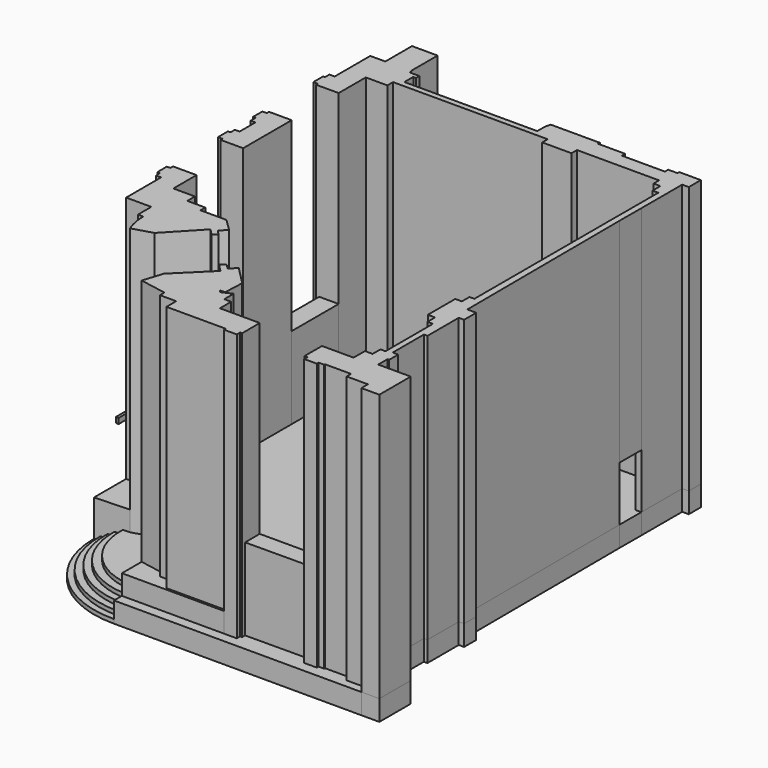
from build123d import *

# Parameters (mm, degrees)
F1_DEPTH      = 9800
F0_W          = 4864.5615577698
F0_H          = 206.8319521715
F2_START      = 2000
F2_DEPTH      = 7800
F3_DEPTH      = 730
F3_DEPTH_BACK = 750
F4_DEPTH      = 2800
F0_W_2        = 366.9002056122
F0_H_2        = 2132.168845481
F0_W_3        = 154.331445694
F0_W_4        = 212.5687599182
F0_W_5        = 342.2532081604
F0_H_3        = 2150.8503360921
F0_W_6        = 172.8549003601
F0_W_7        = 200.4117965698
F5_DEPTH      = 750
F6_START      = -150
F6_DEPTH      = 600
F7_START      = -300
F7_DEPTH      = 450
F8_START      = -450
F8_DEPTH      = 300
F9_START      = -600
F9_DEPTH      = 150
F10_DEPTH     = 3000
F12_W         = 7000
F12_H         = 200
F13_DEPTH     = 100
F14_R         = 253.1505474525
F15_DEPTH     = 1800


with BuildPart() as f1:
    # F0 (on Top) → F1 (new body)
    with BuildSketch(Plane.XY):
        with BuildLine():
            Line((8390.4028525727, 2896.5206632115), (7940.039693393, 3339.2489442326))
            Line((7940.039693393, 3339.2489442326), (6987.7205481903, 3339.2489442326))
            Line((6987.7205481903, 3339.2489442326), (6987.7205481903, 3558.5393704603))
            Line((6987.7205481903, 3558.5393704603), (6329.7600746155, 3558.5393704603))
            Line((6329.7600746155, 3558.5393704603), (6329.7600746155, 3909.2600144575))
            Line((6329.7600746155, 3909.2600144575), (5538.1336212158, 3909.2600144575))
            Line((5538.1336212158, 3909.2600144575), (5538.1336212158, 4971.1712833412))
            Line((5538.1336212158, 4971.1712833412), (5171.2334156036, 4971.1712833412))
            Line((5171.2334156036, 4971.1712833412), (5016.9019699097, 4971.1712833412))
            Line((5016.9019699097, 4971.1712833412), (4804.3332099915, 4971.1712833412))
            Line((4804.3332099915, 4971.1712833412), (4676.3634681702, 4971.1712833412))
            Line((4676.3634681702, 4971.1712833412), (4676.3634681702, 4850.8997164537))
            Line((4676.3634681702, 4850.8997164537), (4546.0958480835, 4850.8997164537))
            Line((4546.0958480835, 4850.8997164537), (4546.0958480835, 4420.0390811927))
            Line((4546.0958480835, 4420.0390811927), (4644.8583602905, 4420.0390811927))
            Line((4644.8583602905, 4420.0390811927), (4644.8583602905, 4229.7711372375))
            Line((4644.8583602905, 4229.7711372375), (4835.2494239807, 4229.7711372375))
            Line((4835.2494239807, 4229.7711372375), (4835.2494239807, 2626.4770030975))
            Line((4835.2494239807, 2626.4770030975), (5757.143497467, 2626.4770030975))
            Line((5757.143497467, 2626.4770030975), (5757.143497467, 2012.3040676117))
            Line((5757.143497467, 2012.3040676117), (5947.5092887878, 2012.3040676117))
            ThreePointArc((5947.5092887878, 2012.3040676117), (5992.5931204612, 1601.8080349278), (6110.9477729288, 1206.1671359211))
            Line((6110.9477729288, 1206.1671359211), (6839.3669128418, 1424.0067005157))
            Line((6839.3669128418, 1424.0067005157), (7948.8120079041, 2597.5522994995))
            Line((7948.8120079041, 2597.5522994995), (8010.4625259152, 2533.099484609))
            Line((8010.4625259152, 2533.099484609), (8155.1715442271, 2671.5168051709))
            Line((8155.1715442271, 2671.5168051709), (8390.4028525727, 2896.5206632115))
        make_face()
        Polygon((8318.0811700354, 2501.2021947697), (8155.1715442271, 2671.5168051709), (8010.4625259152, 2533.099484609), (8175.5933624414, 2360.4626993445), align=None)
    extrude(amount=F1_DEPTH)


with BuildPart() as f1b:
    # F0 (on Top) → F1, piece 2 (new body)
    with BuildSketch(Plane.XY):
        Polygon((5171.2334156036, 7103.3401288221), (5538.1336212158, 7103.3401288221), (5538.1336212158, 9326.2376584242), (5195.8804130554, 9326.2376584242), (5023.0255126953, 9326.2376584242), (4822.6137161255, 9326.2376584242), (4706.4251899719, 9326.2376584242), (4706.4251899719, 9225.9361946481), (4546.0958480835, 9225.9361946481), (4546.0958480835, 8795.1182157243), (4640.9873962402, 8795.1182157243), (4640.9873962402, 8570.7567960466), (4814.5852088928, 8570.7567960466), (4814.5852088928, 7846.2518483842), (4639.1639709473, 7846.2518483842), (4639.1639709473, 7645.8400518144), (4546.0958480835, 7645.8400518144), (4546.0958480835, 7191.3041867445), (4706.4251899719, 7191.3041867445), (4706.4251899719, 7103.3401288221), (4804.3332099915, 7103.3401288221), (5016.9019699097, 7103.3401288221), align=None)
    extrude(amount=F1_DEPTH)


with BuildPart() as f1c:
    # F0 (on Top) → F1, piece 3 (new body)
    with BuildSketch(Plane.XY):
        Polygon((5195.8804130554, 11477.0879945163), (5538.1336212158, 11477.0879945163), (5538.1336212158, 12718.5888089369), (6328.5875320435, 12718.5888089369), (6328.5875320435, 12979.1240491102), (6579.1020393372, 12979.1240491102), (6579.1020393372, 13185.9560012817), (6579.1020393372, 13590.3796948622), (6679.3084144592, 13590.3796948622), (6679.3084144592, 13743.2192050389), (6323.81772995, 13743.2192050389), (6323.81772995, 13838.4149753025), (6296.2608337402, 13838.4149753025), (6296.2608337402, 15059.0704165867), (5357.4075698853, 15059.0704165867), (5357.4075698853, 13838.4149753025), (4806.2753677368, 13838.4149753025), (4806.2753677368, 12207.3677264622), (4616.2400245667, 12207.3677264622), (4616.2400245667, 12006.9559298924), (4546.0958480835, 12006.9559298924), (4546.0958480835, 11556.0431338342), (4706.4251899719, 11556.0431338342), (4706.4251899719, 11477.0879945163), (4822.6137161255, 11477.0879945163), (5023.0255126953, 11477.0879945163), align=None)
        with Locations((9011.382818222, 13082.540025196)):
            Rectangle(F0_W, F0_H)
        Polygon((11443.6635971069, 13185.9560012817), (11443.6635971069, 12979.1240491102), (11992.54322052, 12979.1240491102), (11992.54322052, 12727.0231246948), (13064.7459030151, 12727.0231246948), (13064.7459030151, 12979.1240491102), (16070.9228515625, 12979.1240491102), (16070.9228515625, 12727.0231246948), (16321.4359283447, 12727.0231246948), (16321.4359283447, 12366.2815093994), (16531.867980957, 12366.2815093994), (16531.867980957, 11314.1202926636), (16752.3212432861, 11314.1202926636), (16752.3212432861, 13185.9560012817), (16992.8150177002, 13185.9560012817), (16992.8150177002, 13739.1023635864), (16201.1890411377, 13739.1023635864), (16201.1890411377, 13658.9374542236), (15860.4898452759, 13658.9374542236), (15860.4898452759, 13508.6288452148), (14287.257194519, 13508.6288452148), (14287.257194519, 13658.9374542236), (13295.2194213867, 13658.9374542236), (13295.2194213867, 13739.1023635864), (11495.4862594604, 13739.1023635864), (11443.6635971069, 13556.6558837891), align=None)
    extrude(amount=F1_DEPTH)



with BuildPart() as f1d:
    # F0 (on Top) → F1, piece 4 (new body)
    with BuildSketch(Plane.XY):
        Polygon((17458.3015441895, -2084.8836898804), (17458.3015441895, -2384.4513893127), (18116.828918457, -2384.4513893127), (18116.828918457, -946.4971423149), (16924.3793487549, -946.4971423149), (16924.3793487549, -515.6118869781), (16984.5027923584, -515.6118869781), (16984.5027923584, -104.7678515315), (16784.0919494629, -104.7678515315), (16784.0919494629, 1320.7347393036), (16914.1807556152, 1320.7347393036), (16914.1807556152, 2753.9772987366), (17110.4774475098, 2753.9772987366), (17110.4774475098, 3310.1196289062), (16784.0919494629, 3310.1196289062), (16749.4583129883, 10318.6321258545), (16529.0050506592, 10318.6321258545), (16529.0050506592, 3949.7368335724), (16348.3219146729, 3949.7368335724), (16348.3219146729, 3602.5412082672), (16107.4104309082, 3602.5412082672), (16107.4104309082, 2348.3486175537), (16371.5972900391, 2348.3486175537), (16371.5972900391, 2000.5106925964), (16571.7658996582, 2000.5106925964), (16571.7658996582, -172.0592528582), (16387.3424530029, -172.0592528582), (16387.3424530029, -531.3978791237), (16107.4104309082, -531.3978791237), (16107.4104309082, -1052.1912574768), (14950.7637023926, -1052.1912574768), (14950.7637023926, -1344.4619244273), (14950.7637023926, -1511.5863084793), (14950.7637023926, -1712.9493697641), (14950.7637023926, -1860.01932621), (15058.1789016724, -1860.01932621), (15058.1789016724, -1999.9604225159), (15524.05834198, -1999.9604225159), (15524.05834198, -1918.4757471085), (15724.2269515991, -1918.4757471085), (15724.2269515991, -1883.047580719), (16678.1482696533, -1883.047580719), (16678.1482696533, -2084.8836898804), align=None)
    extrude(amount=F1_DEPTH)


with BuildPart() as f1e:
    # F0 (on Top) → F1, piece 5 (new body)
    with BuildSketch(Plane.XY):
        Polygon((9779.6468734741, 762.6244425774), (8624.6900558472, -378.161162138), (8390.8643722534, -1107.9804897308), (9367.6653263956, -1285.0561902172), (9368.6809539795, -1490.580049064), (9961.6676352145, -1490.580049064), (9963.8738632202, -1937.0355219255), (12124.6039412744, -1937.0355219255), (12124.9885559082, -2014.866692479), (12600.4909252113, -2014.866692479), (12599.7257232666, -1860.01932621), (12674.5738235881, -1860.01932621), (12673.9026556998, -1724.2008268784), (12672.8519885372, -1511.5863084793), (12672.0817630936, -1355.7223797609), (12670.581817627, -1052.1912574768), (11213.5039462497, -1052.1912574768), (11210.9432220459, -533.9994240262), (10957.9822050814, -533.9994240262), (10955.8610916138, -104.7678515315), (10588.4771347046, -271.6313302517), (10517.0803070068, -183.9511841536), (10707.4718475342, -183.9511841536), (10739.1991786456, 560.1845255221), (10076.0921080068, 1231.5289296636), (9847.5538803457, 1005.7948448355), (9691.6052791319, 851.7597184784), align=None)
        Polygon((9504.0505400187, 1041.644324071), (9691.6052791319, 851.7597184784), (9847.5538803457, 1005.7948448355), (9659.9991412325, 1195.6794504281), align=None)
    extrude(amount=F1_DEPTH)


with BuildPart() as f1c_1:
    add(f1c.part)

    add(f1d.part)  # F2 merges F1d
    # F0 (on Top) → F2 (join)
    with BuildSketch(Plane.XY.offset(F2_START)):
        Polygon((16752.3212432861, 11314.1202926636), (16531.867980957, 11314.1202926636), (16529.0050506592, 10318.6321258545), (16749.4583129883, 10318.6321258545), align=None)
    extrude(amount=F2_DEPTH)


with BuildPart() as f3:
    # F0 (on Top) → F3 (new body, two sides)
    with BuildSketch(Plane.XY) as f3_sk:
        with BuildLine():
            Line((5855.5335053998, 1196.4664389317), (6110.9477729288, 1206.1671359211))
            ThreePointArc((6110.9477729288, 1206.1671359211), (5992.5931204612, 1601.8080349278), (5947.5092887878, 2012.3040676117))
            Line((5947.5092887878, 2012.3040676117), (5757.143497467, 2012.3040676117))
            Line((5757.143497467, 2012.3040676117), (5757.143497467, 2626.4770030975))
            Line((5757.143497467, 2626.4770030975), (4835.2494239807, 2626.4770030975))
            Line((4835.2494239807, 2626.4770030975), (4835.2494239807, 2295.9363460541))
            Line((4835.2494239807, 2295.9363460541), (4835.2494239807, 1157.7157974243))
            Line((4835.2494239807, 1157.7157974243), (5065.7572075541, 1166.470539999))
            Line((5065.7572075541, 1166.470539999), (5314.5824427739, 1175.9209839132))
            Line((5314.5824427739, 1175.9209839132), (5563.6743045651, 1185.3815543705))
            Line((5563.6743045651, 1185.3815543705), (5855.5335053998, 1196.4664389317))
        make_face()
    extrude(amount=F3_DEPTH)
    extrude(f3_sk.sketch, amount=-F3_DEPTH_BACK)


with BuildPart() as f3b:
    # F0 (on Top) → F3, piece 2 (new body, two sides)
    with BuildSketch(Plane.XY) as f3_2_sk:
        Polygon((9367.6653263956, -1285.0561902172), (8390.8643722534, -1107.9804897308), (8390.8643722534, -1329.4829130173), (8390.8643722534, -1621.3526725769), (8390.8643722534, -1888.9987468719), (8390.8643722534, -2011.3775971252), (12124.9885559082, -2014.866692479), (12124.6039412744, -1937.0355219255), (9963.8738632202, -1937.0355219255), (9961.6676352145, -1490.580049064), (9368.6809539795, -1490.580049064), align=None)
    extrude(amount=F3_DEPTH)
    extrude(f3_2_sk.sketch, amount=-F3_DEPTH_BACK)


with BuildPart() as f4:
    # F0 (on Top) → F4 (new body)
    with BuildSketch(Plane.XY):
        Polygon((8853.2683259252, 440.7643057013), (9489.7212982178, 1069.4080591202), (9464.7699562199, 1094.2656429276), (8828.5188245168, 465.821253533), align=None)
    extrude(amount=F4_DEPTH)


with BuildPart() as f4b:
    # F0 (on Top) → F4, piece 2 (new body)
    with BuildSketch(Plane.XY):
        Polygon((8251.9132564561, 2304.6191271527), (8208.0926895142, 2343.4784412384), (7569.2801475525, 1709.6762657166), (7610.446964006, 1668.1840151709), align=None)
    extrude(amount=F4_DEPTH)


with BuildPart() as f5:
    # F0 (on Top) → F5 (new body, through all)
    with BuildSketch(Plane.XY):
        with BuildLine():
            Line((6987.7205481903, 3339.2489442326), (7940.039693393, 3339.2489442326))
            Line((7940.039693393, 3339.2489442326), (8390.4028525727, 2896.5206632115))
            Line((8390.4028525727, 2896.5206632115), (8155.1715442271, 2671.5168051709))
            Line((8155.1715442271, 2671.5168051709), (8318.0811700354, 2501.2021947697))
            Line((8318.0811700354, 2501.2021947697), (8175.5933624414, 2360.4626993445))
            Line((8175.5933624414, 2360.4626993445), (8010.4625259152, 2533.099484609))
            Line((8010.4625259152, 2533.099484609), (7948.8120079041, 2597.5522994995))
            Line((7948.8120079041, 2597.5522994995), (6839.3669128418, 1424.0067005157))
            ThreePointArc((6839.3669128418, 1424.0067005157), (7508.6030183957, 301.5856432967), (8624.6900558472, -378.161162138))
            Line((8624.6900558472, -378.161162138), (9779.6468734741, 762.6244425774))
            Line((9779.6468734741, 762.6244425774), (9691.6052791319, 851.7597184784))
            Line((9691.6052791319, 851.7597184784), (9504.0505400187, 1041.644324071))
            Line((9504.0505400187, 1041.644324071), (9659.9991412325, 1195.6794504281))
            Line((9659.9991412325, 1195.6794504281), (9847.5538803457, 1005.7948448355))
            Line((9847.5538803457, 1005.7948448355), (10076.0921080068, 1231.5289296636))
            Line((10076.0921080068, 1231.5289296636), (10739.1991786456, 560.1845255221))
            Line((10739.1991786456, 560.1845255221), (10707.4718475342, -183.9511841536))
            Line((10707.4718475342, -183.9511841536), (10517.0803070068, -183.9511841536))
            Line((10517.0803070068, -183.9511841536), (10588.4771347046, -271.6313302517))
            Line((10588.4771347046, -271.6313302517), (10955.8610916138, -104.7678515315))
            Line((10955.8610916138, -104.7678515315), (10957.9822050814, -533.9994240262))
            Line((10957.9822050814, -533.9994240262), (11210.9432220459, -533.9994240262))
            Line((11210.9432220459, -533.9994240262), (11213.5039462497, -1052.1912574768))
            Line((11213.5039462497, -1052.1912574768), (12670.581817627, -1052.1912574768))
            Line((12670.581817627, -1052.1912574768), (14950.7637023926, -1052.1912574768))
            Line((14950.7637023926, -1052.1912574768), (16107.4104309082, -1052.1912574768))
            Line((16107.4104309082, -1052.1912574768), (16107.4104309082, -531.3978791237))
            Line((16107.4104309082, -531.3978791237), (16387.3424530029, -531.3978791237))
            Line((16387.3424530029, -531.3978791237), (16387.3424530029, -172.0592528582))
            Line((16387.3424530029, -172.0592528582), (16571.7658996582, -172.0592528582))
            Line((16571.7658996582, -172.0592528582), (16571.7658996582, 2000.5106925964))
            Line((16571.7658996582, 2000.5106925964), (16371.5972900391, 2000.5106925964))
            Line((16371.5972900391, 2000.5106925964), (16371.5972900391, 2348.3486175537))
            Line((16371.5972900391, 2348.3486175537), (16107.4104309082, 2348.3486175537))
            Line((16107.4104309082, 2348.3486175537), (16107.4104309082, 3602.5412082672))
            Line((16107.4104309082, 3602.5412082672), (16348.3219146729, 3602.5412082672))
            Line((16348.3219146729, 3602.5412082672), (16348.3219146729, 3949.7368335724))
            Line((16348.3219146729, 3949.7368335724), (16529.0050506592, 3949.7368335724))
            Line((16529.0050506592, 3949.7368335724), (16529.0050506592, 10318.6321258545))
            Line((16529.0050506592, 10318.6321258545), (16531.867980957, 11314.1202926636))
            Line((16531.867980957, 11314.1202926636), (16531.867980957, 12366.2815093994))
            Line((16531.867980957, 12366.2815093994), (16321.4359283447, 12366.2815093994))
            Line((16321.4359283447, 12366.2815093994), (16321.4359283447, 12727.0231246948))
            Line((16321.4359283447, 12727.0231246948), (16070.9228515625, 12727.0231246948))
            Line((16070.9228515625, 12727.0231246948), (16070.9228515625, 12979.1240491102))
            Line((16070.9228515625, 12979.1240491102), (13064.7459030151, 12979.1240491102))
            Line((13064.7459030151, 12979.1240491102), (13064.7459030151, 12727.0231246948))
            Line((13064.7459030151, 12727.0231246948), (11992.54322052, 12727.0231246948))
            Line((11992.54322052, 12727.0231246948), (11992.54322052, 12979.1240491102))
            Line((11992.54322052, 12979.1240491102), (11443.6635971069, 12979.1240491102))
            Line((11443.6635971069, 12979.1240491102), (6579.1020393372, 12979.1240491102))
            Line((6579.1020393372, 12979.1240491102), (6328.5875320435, 12979.1240491102))
            Line((6328.5875320435, 12979.1240491102), (6328.5875320435, 12718.5888089369))
            Line((6328.5875320435, 12718.5888089369), (5538.1336212158, 12718.5888089369))
            Line((5538.1336212158, 12718.5888089369), (5538.1336212158, 11477.0879945163))
            Line((5538.1336212158, 11477.0879945163), (5538.1336212158, 9326.2376584242))
            Line((5538.1336212158, 9326.2376584242), (5538.1336212158, 7103.3401288221))
            Line((5538.1336212158, 7103.3401288221), (5538.1336212158, 4971.1712833412))
            Line((5538.1336212158, 4971.1712833412), (5538.1336212158, 3909.2600144575))
            Line((5538.1336212158, 3909.2600144575), (6329.7600746155, 3909.2600144575))
            Line((6329.7600746155, 3909.2600144575), (6329.7600746155, 3558.5393704603))
            Line((6329.7600746155, 3558.5393704603), (6987.7205481903, 3558.5393704603))
            Line((6987.7205481903, 3558.5393704603), (6987.7205481903, 3339.2489442326))
        make_face()
        Polygon((9464.7699562199, 1094.2656429276), (9489.7212982178, 1069.4080591202), (8853.2683259252, 440.7643057013), (8828.5188245168, 465.821253533), align=None, mode=Mode.SUBTRACT)
        Polygon((7569.2801475525, 1709.6762657166), (8208.0926895142, 2343.4784412384), (8251.9132564561, 2304.6191271527), (7610.446964006, 1668.1840151709), align=None, mode=Mode.SUBTRACT)
        Polygon((8251.9132564561, 2304.6191271527), (8208.0926895142, 2343.4784412384), (7569.2801475525, 1709.6762657166), (7610.446964006, 1668.1840151709), align=None)
        Polygon((8318.0811700354, 2501.2021947697), (8155.1715442271, 2671.5168051709), (8010.4625259152, 2533.099484609), (8175.5933624414, 2360.4626993445), align=None)
        with BuildLine():
            Line((8390.4028525727, 2896.5206632115), (7940.039693393, 3339.2489442326))
            Line((7940.039693393, 3339.2489442326), (6987.7205481903, 3339.2489442326))
            Line((6987.7205481903, 3339.2489442326), (6987.7205481903, 3558.5393704603))
            Line((6987.7205481903, 3558.5393704603), (6329.7600746155, 3558.5393704603))
            Line((6329.7600746155, 3558.5393704603), (6329.7600746155, 3909.2600144575))
            Line((6329.7600746155, 3909.2600144575), (5538.1336212158, 3909.2600144575))
            Line((5538.1336212158, 3909.2600144575), (5538.1336212158, 4971.1712833412))
            Line((5538.1336212158, 4971.1712833412), (5171.2334156036, 4971.1712833412))
            Line((5171.2334156036, 4971.1712833412), (5016.9019699097, 4971.1712833412))
            Line((5016.9019699097, 4971.1712833412), (4804.3332099915, 4971.1712833412))
            Line((4804.3332099915, 4971.1712833412), (4676.3634681702, 4971.1712833412))
            Line((4676.3634681702, 4971.1712833412), (4676.3634681702, 4850.8997164537))
            Line((4676.3634681702, 4850.8997164537), (4546.0958480835, 4850.8997164537))
            Line((4546.0958480835, 4850.8997164537), (4546.0958480835, 4420.0390811927))
            Line((4546.0958480835, 4420.0390811927), (4644.8583602905, 4420.0390811927))
            Line((4644.8583602905, 4420.0390811927), (4644.8583602905, 4229.7711372375))
            Line((4644.8583602905, 4229.7711372375), (4835.2494239807, 4229.7711372375))
            Line((4835.2494239807, 4229.7711372375), (4835.2494239807, 2626.4770030975))
            Line((4835.2494239807, 2626.4770030975), (5757.143497467, 2626.4770030975))
            Line((5757.143497467, 2626.4770030975), (5757.143497467, 2012.3040676117))
            Line((5757.143497467, 2012.3040676117), (5947.5092887878, 2012.3040676117))
            ThreePointArc((5947.5092887878, 2012.3040676117), (5992.5931204612, 1601.8080349278), (6110.9477729288, 1206.1671359211))
            Line((6110.9477729288, 1206.1671359211), (6839.3669128418, 1424.0067005157))
            Line((6839.3669128418, 1424.0067005157), (7948.8120079041, 2597.5522994995))
            Line((7948.8120079041, 2597.5522994995), (8010.4625259152, 2533.099484609))
            Line((8010.4625259152, 2533.099484609), (8155.1715442271, 2671.5168051709))
            Line((8155.1715442271, 2671.5168051709), (8390.4028525727, 2896.5206632115))
        make_face()
        Polygon((9779.6468734741, 762.6244425774), (8624.6900558472, -378.161162138), (8390.8643722534, -1107.9804897308), (9367.6653263956, -1285.0561902172), (9368.6809539795, -1490.580049064), (9961.6676352145, -1490.580049064), (9963.8738632202, -1937.0355219255), (12124.6039412744, -1937.0355219255), (12124.9885559082, -2014.866692479), (12600.4909252113, -2014.866692479), (12599.7257232666, -1860.01932621), (12674.5738235881, -1860.01932621), (12673.9026556998, -1724.2008268784), (12672.8519885372, -1511.5863084793), (12672.0817630936, -1355.7223797609), (12670.581817627, -1052.1912574768), (11213.5039462497, -1052.1912574768), (11210.9432220459, -533.9994240262), (10957.9822050814, -533.9994240262), (10955.8610916138, -104.7678515315), (10588.4771347046, -271.6313302517), (10517.0803070068, -183.9511841536), (10707.4718475342, -183.9511841536), (10739.1991786456, 560.1845255221), (10076.0921080068, 1231.5289296636), (9847.5538803457, 1005.7948448355), (9691.6052791319, 851.7597184784), align=None)
        with Locations((5354.6835184097, 6037.2557060816)):
            Rectangle(F0_W_2, F0_H_2)
        with Locations((5094.0676927567, 6037.2557060816)):
            Rectangle(F0_W_3, F0_H_2)
        with Locations((4910.6175899506, 6037.2557060816)):
            Rectangle(F0_W_4, F0_H_2)
        Polygon((5171.2334156036, 7103.3401288221), (5538.1336212158, 7103.3401288221), (5538.1336212158, 9326.2376584242), (5195.8804130554, 9326.2376584242), (5023.0255126953, 9326.2376584242), (4822.6137161255, 9326.2376584242), (4706.4251899719, 9326.2376584242), (4706.4251899719, 9225.9361946481), (4546.0958480835, 9225.9361946481), (4546.0958480835, 8795.1182157243), (4640.9873962402, 8795.1182157243), (4640.9873962402, 8570.7567960466), (4814.5852088928, 8570.7567960466), (4814.5852088928, 7846.2518483842), (4639.1639709473, 7846.2518483842), (4639.1639709473, 7645.8400518144), (4546.0958480835, 7645.8400518144), (4546.0958480835, 7191.3041867445), (4706.4251899719, 7191.3041867445), (4706.4251899719, 7103.3401288221), (4804.3332099915, 7103.3401288221), (5016.9019699097, 7103.3401288221), align=None)
        with Locations((5367.0070171356, 10401.6628264702)):
            Rectangle(F0_W_5, F0_H_3)
        with Locations((5109.4529628754, 10401.6628264702)):
            Rectangle(F0_W_6, F0_H_3)
        with Locations((4922.8196144104, 10401.6628264702)):
            Rectangle(F0_W_7, F0_H_3)
        Polygon((4676.3634681702, 4971.1712833412), (4804.3332099915, 4971.1712833412), (4804.3332099915, 7103.3401288221), (4706.4251899719, 7103.3401288221), (4706.4251899719, 7191.3041867445), (4546.0958480835, 7191.3041867445), (4546.0958480835, 7645.8400518144), (4639.1639709473, 7645.8400518144), (4639.1639709473, 7846.2518483842), (4814.5852088928, 7846.2518483842), (4814.5852088928, 8570.7567960466), (4640.9873962402, 8570.7567960466), (4640.9873962402, 8795.1182157243), (4546.0958480835, 8795.1182157243), (4546.0958480835, 9225.9361946481), (4706.4251899719, 9225.9361946481), (4706.4251899719, 9326.2376584242), (4822.6137161255, 9326.2376584242), (4822.6137161255, 11477.0879945163), (4706.4251899719, 11477.0879945163), (4706.4251899719, 11556.0431338342), (4546.0958480835, 11556.0431338342), (4546.0958480835, 12006.9559298924), (4616.2400245667, 12006.9559298924), (4616.2400245667, 12207.3677264622), (4806.2753677368, 12207.3677264622), (4806.2753677368, 13838.4149753025), (5357.4075698853, 13838.4149753025), (5357.4075698853, 15059.0704165867), (5251.4958381653, 15059.0704165867), (5251.4958381653, 14151.0353088379), (4505.7363510132, 14151.0353088379), (4505.7363510132, 2295.9363460541), (4835.2494239807, 2295.9363460541), (4835.2494239807, 2626.4770030975), (4835.2494239807, 4229.7711372375), (4644.8583602905, 4229.7711372375), (4644.8583602905, 4420.0390811927), (4546.0958480835, 4420.0390811927), (4546.0958480835, 4850.8997164537), (4676.3634681702, 4850.8997164537), align=None)
        with BuildLine():
            ThreePointArc((8624.6900558472, -378.161162138), (7508.6030183957, 301.5856432967), (6839.3669128418, 1424.0067005157))
            Line((6839.3669128418, 1424.0067005157), (6110.9477729288, 1206.1671359211))
            Line((6110.9477729288, 1206.1671359211), (5855.5335053998, 1196.4664389317))
            ThreePointArc((5855.5335053998, 1196.4664389317), (6569.5049147976, -622.2587111487), (8390.8643722534, -1329.4829130173))
            Line((8390.8643722534, -1329.4829130173), (8390.8643722534, -1107.9804897308))
            Line((8390.8643722534, -1107.9804897308), (8624.6900558472, -378.161162138))
        make_face()
        Polygon((12670.581817627, -1052.1912574768), (12672.0817630936, -1355.7223797609), (14950.7637023926, -1344.4619244273), (14950.7637023926, -1052.1912574768), align=None)
        Polygon((12672.0817630936, -1355.7223797609), (12672.8519885372, -1511.5863084793), (14950.7637023926, -1511.5863084793), (14950.7637023926, -1344.4619244273), align=None)
        Polygon((12672.8519885372, -1511.5863084793), (12673.9026556998, -1724.2008268784), (14950.7637023926, -1712.9493697641), (14950.7637023926, -1511.5863084793), align=None)
        Polygon((8390.8643722534, -2011.3775971252), (8390.8643722534, -2141.2446498871), (8390.8643722534, -2375.9789466858), (17458.3015441895, -2384.4513893127), (17458.3015441895, -2084.8836898804), (16678.1482696533, -2084.8836898804), (16678.1482696533, -1883.047580719), (15724.2269515991, -1883.047580719), (15724.2269515991, -1918.4757471085), (15524.05834198, -1918.4757471085), (15524.05834198, -1999.9604225159), (15058.1789016724, -1999.9604225159), (15058.1789016724, -1860.01932621), (14950.7637023926, -1860.01932621), (14950.7637023926, -1712.9493697641), (12673.9026556998, -1724.2008268784), (12674.5738235881, -1860.01932621), (12599.7257232666, -1860.01932621), (12600.4909252113, -2014.866692479), (12124.9885559082, -2014.866692479), align=None)
        Polygon((17458.3015441895, -2084.8836898804), (17458.3015441895, -2384.4513893127), (18116.828918457, -2384.4513893127), (18116.828918457, -946.4971423149), (16924.3793487549, -946.4971423149), (16924.3793487549, -515.6118869781), (16984.5027923584, -515.6118869781), (16984.5027923584, -104.7678515315), (16784.0919494629, -104.7678515315), (16784.0919494629, 1320.7347393036), (16914.1807556152, 1320.7347393036), (16914.1807556152, 2753.9772987366), (17110.4774475098, 2753.9772987366), (17110.4774475098, 3310.1196289062), (16784.0919494629, 3310.1196289062), (16749.4583129883, 10318.6321258545), (16529.0050506592, 10318.6321258545), (16529.0050506592, 3949.7368335724), (16348.3219146729, 3949.7368335724), (16348.3219146729, 3602.5412082672), (16107.4104309082, 3602.5412082672), (16107.4104309082, 2348.3486175537), (16371.5972900391, 2348.3486175537), (16371.5972900391, 2000.5106925964), (16571.7658996582, 2000.5106925964), (16571.7658996582, -172.0592528582), (16387.3424530029, -172.0592528582), (16387.3424530029, -531.3978791237), (16107.4104309082, -531.3978791237), (16107.4104309082, -1052.1912574768), (14950.7637023926, -1052.1912574768), (14950.7637023926, -1344.4619244273), (14950.7637023926, -1511.5863084793), (14950.7637023926, -1712.9493697641), (14950.7637023926, -1860.01932621), (15058.1789016724, -1860.01932621), (15058.1789016724, -1999.9604225159), (15524.05834198, -1999.9604225159), (15524.05834198, -1918.4757471085), (15724.2269515991, -1918.4757471085), (15724.2269515991, -1883.047580719), (16678.1482696533, -1883.047580719), (16678.1482696533, -2084.8836898804), align=None)
        Polygon((16752.3212432861, 11314.1202926636), (16531.867980957, 11314.1202926636), (16529.0050506592, 10318.6321258545), (16749.4583129883, 10318.6321258545), align=None)
        Polygon((11443.6635971069, 13185.9560012817), (11443.6635971069, 12979.1240491102), (11992.54322052, 12979.1240491102), (11992.54322052, 12727.0231246948), (13064.7459030151, 12727.0231246948), (13064.7459030151, 12979.1240491102), (16070.9228515625, 12979.1240491102), (16070.9228515625, 12727.0231246948), (16321.4359283447, 12727.0231246948), (16321.4359283447, 12366.2815093994), (16531.867980957, 12366.2815093994), (16531.867980957, 11314.1202926636), (16752.3212432861, 11314.1202926636), (16752.3212432861, 13185.9560012817), (16992.8150177002, 13185.9560012817), (16992.8150177002, 13739.1023635864), (16201.1890411377, 13739.1023635864), (16201.1890411377, 13658.9374542236), (15860.4898452759, 13658.9374542236), (15860.4898452759, 13508.6288452148), (14287.257194519, 13508.6288452148), (14287.257194519, 13658.9374542236), (13295.2194213867, 13658.9374542236), (13295.2194213867, 13739.1023635864), (11495.4862594604, 13739.1023635864), (11443.6635971069, 13556.6558837891), align=None)
        with Locations((9011.382818222, 13082.540025196)):
            Rectangle(F0_W, F0_H)
        Polygon((5195.8804130554, 11477.0879945163), (5538.1336212158, 11477.0879945163), (5538.1336212158, 12718.5888089369), (6328.5875320435, 12718.5888089369), (6328.5875320435, 12979.1240491102), (6579.1020393372, 12979.1240491102), (6579.1020393372, 13185.9560012817), (6579.1020393372, 13590.3796948622), (6679.3084144592, 13590.3796948622), (6679.3084144592, 13743.2192050389), (6323.81772995, 13743.2192050389), (6323.81772995, 13838.4149753025), (6296.2608337402, 13838.4149753025), (6296.2608337402, 15059.0704165867), (5357.4075698853, 15059.0704165867), (5357.4075698853, 13838.4149753025), (4806.2753677368, 13838.4149753025), (4806.2753677368, 12207.3677264622), (4616.2400245667, 12207.3677264622), (4616.2400245667, 12006.9559298924), (4546.0958480835, 12006.9559298924), (4546.0958480835, 11556.0431338342), (4706.4251899719, 11556.0431338342), (4706.4251899719, 11477.0879945163), (4822.6137161255, 11477.0879945163), (5023.0255126953, 11477.0879945163), align=None)
        Polygon((9504.0505400187, 1041.644324071), (9691.6052791319, 851.7597184784), (9847.5538803457, 1005.7948448355), (9659.9991412325, 1195.6794504281), align=None)
        Polygon((8853.2683259252, 440.7643057013), (9489.7212982178, 1069.4080591202), (9464.7699562199, 1094.2656429276), (8828.5188245168, 465.821253533), align=None)
    extrude(amount=-F5_DEPTH)

    # F0 (on Top) → F6 (join)
    with BuildSketch(Plane.XY.offset(F6_START)):
        with BuildLine():
            ThreePointArc((8390.8643722534, -1329.4829130173), (6569.5049147976, -622.2587111487), (5855.5335053998, 1196.4664389317))
            Line((5855.5335053998, 1196.4664389317), (5563.6743045651, 1185.3815543705))
            ThreePointArc((5563.6743045651, 1185.3815543705), (6369.3895025015, -830.2957015906), (8390.8643722534, -1621.3526725769))
            Line((8390.8643722534, -1621.3526725769), (8390.8643722534, -1329.4829130173))
        make_face()
    extrude(amount=-F6_DEPTH)

    # F0 (on Top) → F7 (join)
    with BuildSketch(Plane.XY.offset(F7_START)):
        with BuildLine():
            ThreePointArc((8390.8643722534, -1621.3526725769), (6369.3895025015, -830.2957015906), (5563.6743045651, 1185.3815543705))
            Line((5563.6743045651, 1185.3815543705), (5314.5824427739, 1175.9209839132))
            ThreePointArc((5314.5824427739, 1175.9209839132), (6199.9333473698, -1011.7489496563), (8390.8643722534, -1888.9987468719))
            Line((8390.8643722534, -1888.9987468719), (8390.8643722534, -1621.3526725769))
        make_face()
    extrude(amount=-F7_DEPTH)

    # F0 (on Top) → F8 (join)
    with BuildSketch(Plane.XY.offset(F8_START)):
        with BuildLine():
            ThreePointArc((8390.8643722534, -1888.9987468719), (6199.9333473698, -1011.7489496563), (5314.5824427739, 1175.9209839132))
            Line((5314.5824427739, 1175.9209839132), (5065.7572075541, 1166.470539999))
            ThreePointArc((5065.7572075541, 1166.470539999), (6026.8244693673, -1192.5617923236), (8390.8643722534, -2141.2446498871))
            Line((8390.8643722534, -2141.2446498871), (8390.8643722534, -2011.3775971252))
            Line((8390.8643722534, -2011.3775971252), (8390.8643722534, -1888.9987468719))
        make_face()
    extrude(amount=-F8_DEPTH)

    # F0 (on Top) → F9 (join)
    with BuildSketch(Plane.XY.offset(F9_START)):
        with BuildLine():
            ThreePointArc((8390.8643722534, -2141.2446498871), (6026.8244693673, -1192.5617923236), (5065.7572075541, 1166.470539999))
            Line((5065.7572075541, 1166.470539999), (4835.2494239807, 1157.7157974243))
            ThreePointArc((4835.2494239807, 1157.7157974243), (5878.0024971754, -1348.7456627288), (8390.8643722534, -2375.9789466858))
            Line((8390.8643722534, -2375.9789466858), (8390.8643722534, -2141.2446498871))
        make_face()
    extrude(amount=-F9_DEPTH)


with BuildPart() as f10:
    # F0 (on Top) → F10 (new body)
    with BuildSketch(Plane.XY):
        Polygon((12670.581817627, -1052.1912574768), (12672.0817630936, -1355.7223797609), (14950.7637023926, -1344.4619244273), (14950.7637023926, -1052.1912574768), align=None)
        Polygon((12672.0817630936, -1355.7223797609), (12672.8519885372, -1511.5863084793), (14950.7637023926, -1511.5863084793), (14950.7637023926, -1344.4619244273), align=None)
        Polygon((12672.8519885372, -1511.5863084793), (12673.9026556998, -1724.2008268784), (14950.7637023926, -1712.9493697641), (14950.7637023926, -1511.5863084793), align=None)
    extrude(amount=F10_DEPTH)


with BuildPart() as f10b:
    # F0 (on Top) → F10, piece 2 (new body)
    with BuildSketch(Plane.XY):
        with Locations((5354.6835184097, 6037.2557060816)):
            Rectangle(F0_W_2, F0_H_2)
        with Locations((5094.0676927567, 6037.2557060816)):
            Rectangle(F0_W_3, F0_H_2)
        with Locations((4910.6175899506, 6037.2557060816)):
            Rectangle(F0_W_4, F0_H_2)
    extrude(amount=F10_DEPTH)


with BuildPart() as f10c:
    # F0 (on Top) → F10, piece 3 (new body)
    with BuildSketch(Plane.XY):
        with Locations((5367.0070171356, 10401.6628264702)):
            Rectangle(F0_W_5, F0_H_3)
        with Locations((4922.8196144104, 10401.6628264702)):
            Rectangle(F0_W_7, F0_H_3)
        with Locations((5109.4529628754, 10401.6628264702)):
            Rectangle(F0_W_6, F0_H_3)
    extrude(amount=F10_DEPTH)


with BuildPart() as f13:
    # F12 (on face) → F13 (new body)
    with BuildSketch(Plane(origin=(4822.6137161255, 0, 0), x_dir=(0, -1, 0), z_dir=(-1, 0, 0))):
        with Locations((-5799.8386655784, 2725.029706955)):
            Rectangle(F12_W, F12_H)
    extrude(amount=F13_DEPTH)


with BuildPart() as f15:
    # F14 (on face) → F15 (new body)
    with BuildSketch(Plane.XY):
        with Locations((11607.8929901123, 3615.6160831451)):
            Circle(F14_R)
    extrude(amount=F15_DEPTH)


solid = Compound([f1.part, f1b.part, f1e.part, f1c_1.part, f3.part, f3b.part, f4.part, f4b.part, f5.part, f10.part, f10b.part, f10c.part, f13.part, f15.part])
